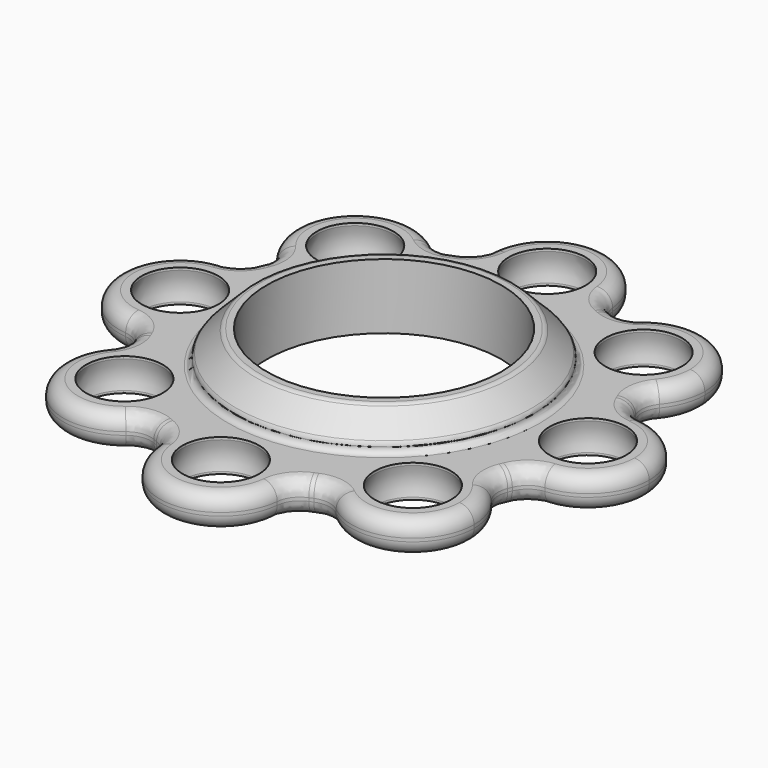
from build123d import *

# Parameters (mm, degrees)
F0_R          = 14.375
F1_DEPTH      = 2
F1_DEPTH_BACK = 2
F2_R          = 3
F3_R          = 1.8
F22_R         = 18.375
F22_R_2       = 14.375
F23_DEPTH     = 4
F24_SIZE      = 2.9
F25_R         = 0.75


with BuildPart() as f1:
    # F0 (on Top) → F1 (new body, two sides)
    with BuildSketch(Plane.XY) as f1_sk:
        with BuildLine():
            ThreePointArc((7.415145, 23.875), (0, 17.5), (-7.415145, 23.875))
            ThreePointArc((-7.415145, 23.875), (-9.567086, 23.096988), (-11.638875, 22.125474))
            ThreePointArc((-11.638875, 22.125474), (-10.552329, 20.018507), (-10.17767, 17.67767))
            ThreePointArc((-10.17767, 17.67767), (-14.294515, 10.984071), (-22.125474, 11.638875))
            ThreePointArc((-22.125474, 11.638875), (-23.096988, 9.567086), (-23.875, 7.415145))
            ThreePointArc((-23.875, 7.415145), (-19.312843, 4.889402), (-17.5, 0))
            ThreePointArc((-17.5, 0), (-19.312843, -4.889402), (-23.875, -7.415145))
            ThreePointArc((-23.875, -7.415145), (-23.096988, -9.567086), (-22.125474, -11.638875))
            ThreePointArc((-22.125474, -11.638875), (-14.294515, -10.984071), (-10.17767, -17.67767))
            ThreePointArc((-10.17767, -17.67767), (-10.552329, -20.018507), (-11.638875, -22.125474))
            ThreePointArc((-11.638875, -22.125474), (-9.567086, -23.096988), (-7.415145, -23.875))
            ThreePointArc((-7.415145, -23.875), (0, -17.5), (7.415145, -23.875))
            ThreePointArc((7.415145, -23.875), (9.567086, -23.096988), (11.638875, -22.125474))
            ThreePointArc((11.638875, -22.125474), (12.374369, -12.374369), (22.125474, -11.638875))
            ThreePointArc((22.125474, -11.638875), (23.096988, -9.567086), (23.875, -7.415145))
            ThreePointArc((23.875, -7.415145), (17.5, 0), (23.875, 7.415145))
            ThreePointArc((23.875, 7.415145), (23.096988, 9.567086), (22.125474, 11.638875))
            ThreePointArc((22.125474, 11.638875), (12.374369, 12.374369), (11.638875, 22.125474))
            ThreePointArc((11.638875, 22.125474), (9.567086, 23.096988), (7.415145, 23.875))
        make_face()
        Circle(F0_R, mode=Mode.SUBTRACT)
        with BuildLine():
            ThreePointArc((-20.673956, -14.056583), (-21.433831, -12.868212), (-22.125474, -11.638875))
            ThreePointArc((-22.125474, -11.638875), (-22.98097, -22.98097), (-11.638875, -22.125474))
            ThreePointArc((-11.638875, -22.125474), (-12.868212, -21.433831), (-14.056583, -20.673956))
            ThreePointArc((-14.056583, -20.673956), (-21.001071, -21.001071), (-20.673956, -14.056583))
        make_face()
        with BuildLine():
            ThreePointArc((-10.17767, -17.67767), (-14.294515, -10.984071), (-22.125474, -11.638875))
            ThreePointArc((-22.125474, -11.638875), (-21.433831, -12.868212), (-20.673956, -14.056583))
            ThreePointArc((-20.673956, -14.056583), (-15.676738, -13.424874), (-12.97767, -17.67767))
            ThreePointArc((-12.97767, -17.67767), (-13.255617, -19.269978), (-14.056583, -20.673956))
            ThreePointArc((-14.056583, -20.673956), (-12.868212, -21.433831), (-11.638875, -22.125474))
            ThreePointArc((-11.638875, -22.125474), (-10.552329, -20.018507), (-10.17767, -17.67767))
        make_face()
        with BuildLine():
            ThreePointArc((-17.5, 0), (-19.312843, 4.889402), (-23.875, 7.415145))
            ThreePointArc((-23.875, 7.415145), (-24.255207, 6.056808), (-24.5582, 4.679189))
            ThreePointArc((-24.5582, 4.679189), (-21.523906, 3.163348), (-20.3, 0))
            ThreePointArc((-20.3, 0), (-21.523906, -3.163348), (-24.5582, -4.679189))
            ThreePointArc((-24.5582, -4.679189), (-24.255207, -6.056808), (-23.875, -7.415145))
            ThreePointArc((-23.875, -7.415145), (-19.312843, -4.889402), (-17.5, 0))
        make_face()
        with BuildLine():
            ThreePointArc((-24.5582, 4.679189), (-24.255207, 6.056808), (-23.875, 7.415145))
            ThreePointArc((-23.875, 7.415145), (-32.5, 0), (-23.875, -7.415145))
            ThreePointArc((-23.875, -7.415145), (-24.255207, -6.056808), (-24.5582, -4.679189))
            ThreePointArc((-24.5582, -4.679189), (-29.7, 0), (-24.5582, 4.679189))
        make_face()
        with BuildLine():
            ThreePointArc((-14.056583, 20.673956), (-12.868212, 21.433831), (-11.638875, 22.125474))
            ThreePointArc((-11.638875, 22.125474), (-22.98097, 22.98097), (-22.125474, 11.638875))
            ThreePointArc((-22.125474, 11.638875), (-21.433831, 12.868212), (-20.673956, 14.056583))
            ThreePointArc((-20.673956, 14.056583), (-21.001071, 21.001071), (-14.056583, 20.673956))
        make_face()
        with BuildLine():
            ThreePointArc((-10.17767, 17.67767), (-10.552329, 20.018507), (-11.638875, 22.125474))
            ThreePointArc((-11.638875, 22.125474), (-12.868212, 21.433831), (-14.056583, 20.673956))
            ThreePointArc((-14.056583, 20.673956), (-13.255617, 19.269978), (-12.97767, 17.67767))
            ThreePointArc((-12.97767, 17.67767), (-15.676738, 13.424874), (-20.673956, 14.056583))
            ThreePointArc((-20.673956, 14.056583), (-21.433831, 12.868212), (-22.125474, 11.638875))
            ThreePointArc((-22.125474, 11.638875), (-14.294515, 10.984071), (-10.17767, 17.67767))
        make_face()
        with BuildLine():
            ThreePointArc((-4.679189, 24.5582), (-0.221145, 29.694794), (4.7, 25))
            ThreePointArc((4.7, 25), (4.694794, 24.778855), (4.679189, 24.5582))
            ThreePointArc((4.679189, 24.5582), (6.056808, 24.255207), (7.415145, 23.875))
            ThreePointArc((7.415145, 23.875), (7.478756, 24.435902), (7.5, 25))
            ThreePointArc((7.5, 25), (-0.564098, 32.478756), (-7.415145, 23.875))
            ThreePointArc((-7.415145, 23.875), (-6.056808, 24.255207), (-4.679189, 24.5582))
        make_face()
        with BuildLine():
            ThreePointArc((4.679189, 24.5582), (0, 20.3), (-4.679189, 24.5582))
            ThreePointArc((-4.679189, 24.5582), (-6.056808, 24.255207), (-7.415145, 23.875))
            ThreePointArc((-7.415145, 23.875), (0, 17.5), (7.415145, 23.875))
            ThreePointArc((7.415145, 23.875), (6.056808, 24.255207), (4.679189, 24.5582))
        make_face()
        with BuildLine():
            ThreePointArc((25.17767, 17.67767), (20.018507, 24.80301), (11.638875, 22.125474))
            ThreePointArc((11.638875, 22.125474), (12.868212, 21.433831), (14.056583, 20.673956))
            ThreePointArc((14.056583, 20.673956), (19.269978, 22.099723), (22.37767, 17.67767))
            ThreePointArc((22.37767, 17.67767), (21.930466, 15.676738), (20.673956, 14.056583))
            ThreePointArc((20.673956, 14.056583), (21.433831, 12.868212), (22.125474, 11.638875))
            ThreePointArc((22.125474, 11.638875), (24.371268, 14.294515), (25.17767, 17.67767))
        make_face()
        with BuildLine():
            ThreePointArc((14.056583, 20.673956), (12.868212, 21.433831), (11.638875, 22.125474))
            ThreePointArc((11.638875, 22.125474), (12.374369, 12.374369), (22.125474, 11.638875))
            ThreePointArc((22.125474, 11.638875), (21.433831, 12.868212), (20.673956, 14.056583))
            ThreePointArc((20.673956, 14.056583), (14.354268, 14.354268), (14.056583, 20.673956))
        make_face()
        with BuildLine():
            ThreePointArc((24.5582, 4.679189), (24.255207, 6.056808), (23.875, 7.415145))
            ThreePointArc((23.875, 7.415145), (17.5, 0), (23.875, -7.415145))
            ThreePointArc((23.875, -7.415145), (24.255207, -6.056808), (24.5582, -4.679189))
            ThreePointArc((24.5582, -4.679189), (20.3, 0), (24.5582, 4.679189))
        make_face()
        with BuildLine():
            ThreePointArc((32.5, 0), (29.889402, 5.687157), (23.875, 7.415145))
            ThreePointArc((23.875, 7.415145), (24.255207, 6.056808), (24.5582, 4.679189))
            ThreePointArc((24.5582, 4.679189), (28.163348, 3.476094), (29.7, 0))
            ThreePointArc((29.7, 0), (28.163348, -3.476094), (24.5582, -4.679189))
            ThreePointArc((24.5582, -4.679189), (24.255207, -6.056808), (23.875, -7.415145))
            ThreePointArc((23.875, -7.415145), (29.889402, -5.687157), (32.5, 0))
        make_face()
        with BuildLine():
            ThreePointArc((25.17767, -17.67767), (24.371268, -14.294515), (22.125474, -11.638875))
            ThreePointArc((22.125474, -11.638875), (21.433831, -12.868212), (20.673956, -14.056583))
            ThreePointArc((20.673956, -14.056583), (21.930466, -15.676738), (22.37767, -17.67767))
            ThreePointArc((22.37767, -17.67767), (19.269978, -22.099723), (14.056583, -20.673956))
            ThreePointArc((14.056583, -20.673956), (12.868212, -21.433831), (11.638875, -22.125474))
            ThreePointArc((11.638875, -22.125474), (20.018507, -24.80301), (25.17767, -17.67767))
        make_face()
        with BuildLine():
            ThreePointArc((20.673956, -14.056583), (21.433831, -12.868212), (22.125474, -11.638875))
            ThreePointArc((22.125474, -11.638875), (12.374369, -12.374369), (11.638875, -22.125474))
            ThreePointArc((11.638875, -22.125474), (12.868212, -21.433831), (14.056583, -20.673956))
            ThreePointArc((14.056583, -20.673956), (14.354268, -14.354268), (20.673956, -14.056583))
        make_face()
        with BuildLine():
            ThreePointArc((-4.679189, -24.5582), (-6.056808, -24.255207), (-7.415145, -23.875))
            ThreePointArc((-7.415145, -23.875), (-0.564098, -32.478756), (7.5, -25))
            ThreePointArc((7.5, -25), (7.478756, -24.435902), (7.415145, -23.875))
            ThreePointArc((7.415145, -23.875), (6.056808, -24.255207), (4.679189, -24.5582))
            ThreePointArc((4.679189, -24.5582), (4.694794, -24.778855), (4.7, -25))
            ThreePointArc((4.7, -25), (-0.221145, -29.694794), (-4.679189, -24.5582))
        make_face()
        with BuildLine():
            ThreePointArc((7.415145, -23.875), (0, -17.5), (-7.415145, -23.875))
            ThreePointArc((-7.415145, -23.875), (-6.056808, -24.255207), (-4.679189, -24.5582))
            ThreePointArc((-4.679189, -24.5582), (0, -20.3), (4.679189, -24.5582))
            ThreePointArc((4.679189, -24.5582), (6.056808, -24.255207), (7.415145, -23.875))
        make_face()
    extrude(amount=F1_DEPTH)
    extrude(f1_sk.sketch, amount=-F1_DEPTH_BACK)

    # F2
    f2_edges = [f1.edges().sort_by_distance(p)[0] for p in [
        (7.415145, -23.875, 0),
        (-23.875, -7.415145, 0),
        (-23.875, 7.415145, 0),
        (7.415145, 23.875, 0),
        (22.125474, 11.638875, 0),
        (-22.125474, 11.638875, 0),
        (-22.125474, -11.638875, 0),
        (-11.638875, 22.125474, 0),
        (-7.415145, 23.875, 0),
        (23.875, 7.415145, 0),
        (11.638875, 22.125474, 0),
        (23.875, -7.415145, 0),
        (11.638875, -22.125474, 0),
        (22.125474, -11.638875, 0),
        (-7.415145, -23.875, 0),
        (-11.638875, -22.125474, 0),
    ]]
    fillet(f2_edges, radius=F2_R)

    # F3
    f3_edges = [f1.edges().sort_by_distance(p)[0] for p in [
        (22.98097, 22.98097, 2),
        (22.98097, 22.98097, -2),
    ]]
    fillet(f3_edges, radius=F3_R)


with BuildPart() as f5:
    # F4 (on Right) → F5 (revolve)
    with BuildSketch(Plane.YZ):
        with BuildLine():
            Line((-25, -5), (-25, 5))
            ThreePointArc((-25, 5), (-30, 0), (-25, -5))
        make_face()
    revolve(axis=Axis((0, -25, -0.930661), (0, 0, -1)))


with BuildPart() as f6:
    # F4 (on Right) → F6 (revolve)
    with BuildSketch(Plane.YZ):
        with BuildLine():
            Line((25, 5), (25, -5))
            ThreePointArc((25, -5), (30, 0), (25, 5))
        make_face()
    revolve(axis=Axis((0, 25, -1.024194), (0, 0, -1)))


with BuildPart() as f1_1:
    add(f1.part)

    # F7: cut F6, F5
    add(f6.part, mode=Mode.SUBTRACT)
    add(f5.part, mode=Mode.SUBTRACT)


with BuildPart() as f9:
    # F8 (on Front) → F9 (revolve)
    with BuildSketch(Plane.XZ):
        with BuildLine():
            Line((-25, -5), (-25, 5))
            ThreePointArc((-25, 5), (-30, 0), (-25, -5))
        make_face()
    revolve(axis=Axis((-25, 0, -1.001059), (0, 0, -1)))


with BuildPart() as f10:
    # F8 (on Front) → F10 (revolve)
    with BuildSketch(Plane.XZ):
        with BuildLine():
            Line((25, 5), (25, -5))
            ThreePointArc((25, -5), (30, 0), (25, 5))
        make_face()
    revolve(axis=Axis((25, 0, -1.00106), (0, 0, -1)))


with BuildPart() as f1_2:
    add(f1_1.part)

    # F11: cut F9, F10
    add(f9.part, mode=Mode.SUBTRACT)
    add(f10.part, mode=Mode.SUBTRACT)


with BuildPart() as f14:
    # F13 (on plane+point) → F14 (revolve)
    with BuildSketch(Plane.XZ.offset(17.67767)):
        with BuildLine():
            Line((-17.67767, -5), (-17.67767, 5))
            ThreePointArc((-17.67767, 5), (-22.67767, 0), (-17.67767, -5))
        make_face()
    revolve(axis=Axis((-17.67767, -17.67767, -2.516819), (0, 0, -1)))


with BuildPart() as f15:
    # F13 (on plane+point) → F15 (revolve)
    with BuildSketch(Plane.XZ.offset(17.67767)):
        with BuildLine():
            Line((17.67767, 5), (17.67767, -5))
            ThreePointArc((17.67767, -5), (22.67767, 0), (17.67767, 5))
        make_face()
    revolve(axis=Axis((17.67767, -17.67767, -2.359518), (0, 0, -1)))


with BuildPart() as f1_3:
    add(f1_2.part)

    # F16: cut F15, F14
    add(f15.part, mode=Mode.SUBTRACT)
    add(f14.part, mode=Mode.SUBTRACT)


with BuildPart() as f19:
    # F18 (on plane+point) → F19 (revolve)
    with BuildSketch(Plane.XZ.offset(-17.67767)):
        with BuildLine():
            Line((17.67767, 5), (17.67767, -5))
            ThreePointArc((17.67767, -5), (22.67767, 0), (17.67767, 5))
        make_face()
    revolve(axis=Axis((17.67767, 17.67767, 0.778604), (0, 0, -1)))


with BuildPart() as f20:
    # F18 (on plane+point) → F20 (revolve)
    with BuildSketch(Plane.XZ.offset(-17.67767)):
        with BuildLine():
            Line((-17.67767, -5), (-17.67767, 5))
            ThreePointArc((-17.67767, 5), (-22.67767, 0), (-17.67767, -5))
        make_face()
    revolve(axis=Axis((-17.67767, 17.67767, 1.557206), (0, 0, -1)))


with BuildPart() as f1_4:
    add(f1_3.part)

    # F21: cut F20, F19
    add(f20.part, mode=Mode.SUBTRACT)
    add(f19.part, mode=Mode.SUBTRACT)

    # F22 (on face) → F23 (join)
    with BuildSketch(Plane.XY.offset(2)):
        Circle(F22_R)
        Circle(F22_R_2, mode=Mode.SUBTRACT)
    extrude(amount=F23_DEPTH)

    # F24
    f24_edges = [f1_4.edges().sort_by_distance(p)[0] for p in [
        (-18.375, 0, 6),
    ]]
    chamfer(f24_edges, length=F24_SIZE)

    # F25
    f25_edges = [f1_4.edges().sort_by_distance(p)[0] for p in [
        (-18.375, 0, 2),
        (-15.475, 0, 6),
        (-18.375, 0, 3.1),
    ]]
    fillet(f25_edges, radius=F25_R)


solid = f1_4.part
